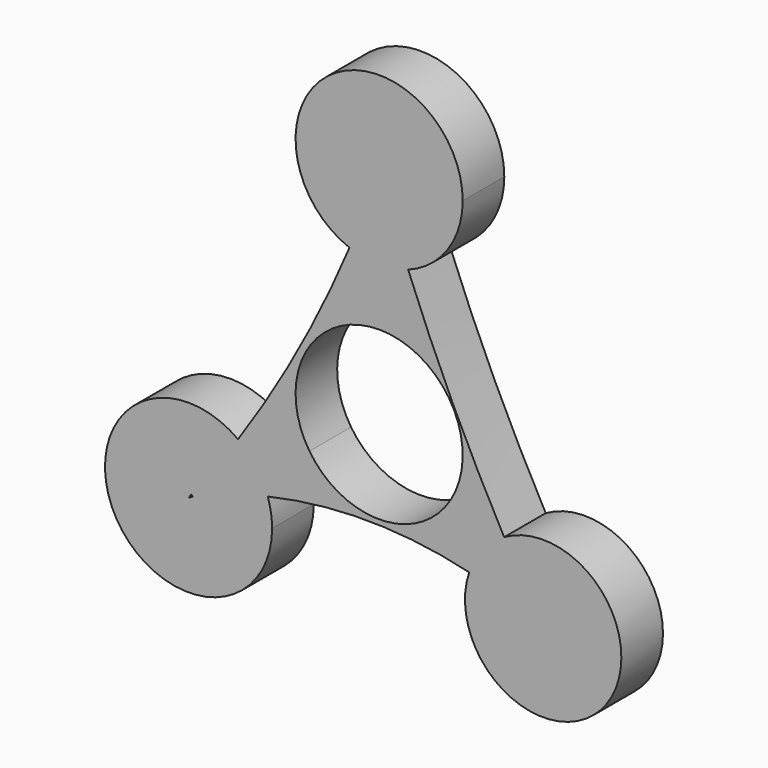
from build123d import *

# Parameters (mm, degrees)
F1_DEPTH = 7


with BuildPart() as f1:
    # F0 (on Front) → F1 (new body)
    with BuildSketch(Plane.XZ):
        with BuildLine():
            ThreePointArc((0, 11.25), (7.9549512883, 7.9549512883), (11.25, 0))
            ThreePointArc((11.25, 0), (10.6496799821, -3.625853869), (8.912788217, -6.8647437096))
            Line((8.912788217, -6.8647437096), (13.7440443636, -10.5858391104))
            ThreePointArc((13.7440443636, -10.5858391104), (15.1532765292, -9.0858880946), (16.8274285565, -7.8888069213))
            ThreePointArc((16.8274285565, -7.8888069213), (9.9384051979, 5.6621865141), (3.902940072, 19.6142912527))
            ThreePointArc((3.902940072, 19.6142912527), (1.9824951191, 19.091630603), (0, 18.9155735821))
            Line((0, 18.9155735821), (0, 11.25))
        make_face()
        with BuildLine():
            ThreePointArc((-9.3763874584, -6.216579303), (-9.9120890119, 5.3209953412), (0, 11.25))
            Line((0, 11.25), (0, 18.9155735821))
            ThreePointArc((0, 18.9155735821), (-2.0297975666, 19.1002031934), (-3.9929710023, 19.6480319218))
            ThreePointArc((-3.9929710023, 19.6480319218), (-10.8071521762, 5.4794924629), (-18.9966353601, -7.9411237916))
            ThreePointArc((-18.9966353601, -7.9411237916), (-17.5117499257, -9.2469886158), (-16.2784463054, -10.7926696541))
            Line((-16.2784463054, -10.7926696541), (-9.3763874584, -6.216579303))
        make_face()
        with BuildLine():
            Line((13.7440443636, -10.5858391104), (8.912788217, -6.8647437096))
            ThreePointArc((8.912788217, -6.8647437096), (-0.3984474102, -11.2429417708), (-9.3763874584, -6.216579303))
            Line((-9.3763874584, -6.216579303), (-16.2784463054, -10.7926696541))
            ThreePointArc((-16.2784463054, -10.7926696541), (-15.5501585, -12.0637421264), (-14.9932083314, -13.4186719648))
            ThreePointArc((-14.9932083314, -13.4186719648), (-1.4222887066, -11.9055225601), (12.1287440927, -13.58748292))
            ThreePointArc((12.1287440927, -13.58748292), (12.8140917314, -12.020845326), (13.7440443636, -10.5858391104))
        make_face()
        with BuildLine():
            Line((0, 30.1655735821), (0, 18.9155735821))
            ThreePointArc((0, 18.9155735821), (1.9824951191, 19.091630603), (3.902940072, 19.6142912527))
            ThreePointArc((3.902940072, 19.6142912527), (1.8909068472, 24.8675299748), (0, 30.1655735821))
        make_face()
        with BuildLine():
            ThreePointArc((-3.9929710023, 19.6480319218), (-2.0297975666, 19.1002031934), (0, 18.9155735821))
            Line((0, 18.9155735821), (0, 30.1655735821))
            ThreePointArc((0, 30.1655735821), (-1.902781485, 24.8712281442), (-3.9929710023, 19.6480319218))
        make_face()
        with BuildLine():
            Line((22.0838300884, -17.009248957), (13.7440443636, -10.5858391104))
            ThreePointArc((13.7440443636, -10.5858391104), (12.8140917314, -12.020845326), (12.1287440927, -13.58748292))
            ThreePointArc((12.1287440927, -13.58748292), (17.1835996068, -15.0734374251), (22.0838300884, -17.009248957))
        make_face()
        with BuildLine():
            ThreePointArc((16.8274285565, -7.8888069213), (15.1532765292, -9.0858880946), (13.7440443636, -10.5858391104))
            Line((13.7440443636, -10.5858391104), (22.0838300884, -17.009248957))
            ThreePointArc((22.0838300884, -17.009248957), (19.4066454, -12.4772589354), (16.8274285565, -7.8888069213))
        make_face()
        with BuildLine():
            Line((-25.1416982942, -16.6690382571), (-16.2784463054, -10.7926696541))
            ThreePointArc((-16.2784463054, -10.7926696541), (-17.5117499257, -9.2469886158), (-18.9966353601, -7.9411237916))
            ThreePointArc((-18.9966353601, -7.9411237916), (-22.0531670318, -12.2727527283), (-25.2533971823, -16.4993260556))
            ThreePointArc((-25.2533971823, -16.4993260556), (-25.19769062, -16.5842761963), (-25.1416982942, -16.6690382571))
        make_face()
        with BuildLine():
            ThreePointArc((-14.9932083314, -13.4186719648), (-15.5501585, -12.0637421264), (-16.2784463054, -10.7926696541))
            Line((-16.2784463054, -10.7926696541), (-25.1416982942, -16.6690382571))
            ThreePointArc((-25.1416982942, -16.6690382571), (-25.1125512398, -16.7129171531), (-25.0833276051, -16.7567450833))
            ThreePointArc((-25.0833276051, -16.7567450833), (-20.114417639, -14.8575280476), (-14.9932083314, -13.4186719648))
        make_face()
        with BuildLine():
            ThreePointArc((11.25, 30.1655735821), (-6.3891148144, 39.425255644), (-3.9929710023, 19.6480319218))
            ThreePointArc((-3.9929710023, 19.6480319218), (-1.902781485, 24.8712281442), (0, 30.1655735821))
            ThreePointArc((0, 30.1655735821), (1.8909068472, 24.8675299748), (3.902940072, 19.6142912527))
            ThreePointArc((3.902940072, 19.6142912527), (9.2322959173, 23.7369491495), (11.25, 30.1655735821))
        make_face()
        with BuildLine():
            ThreePointArc((32.6105684243, -17.009248957), (27.3506819222, -7.8948377444), (16.8274285565, -7.8888069213))
            ThreePointArc((16.8274285565, -7.8888069213), (19.4066454, -12.4772589354), (22.0838300884, -17.009248957))
            ThreePointArc((22.0838300884, -17.009248957), (17.1835996068, -15.0734374251), (12.1287440927, -13.58748292))
            ThreePointArc((12.1287440927, -13.58748292), (20.3492358123, -27.3920907015), (32.6105684243, -17.009248957))
        make_face()
        with BuildLine():
            ThreePointArc((-14.4048337638, -17.009248957), (-14.5529018122, -15.1900164424), (-14.9932083314, -13.4186719648))
            ThreePointArc((-14.9932083314, -13.4186719648), (-20.114417639, -14.8575280476), (-25.0833276051, -16.7567450833))
            ThreePointArc((-25.0833276051, -16.7567450833), (-25.3694186196, -16.8822321528), (-25.6548337638, -17.009248957))
            ThreePointArc((-25.6548337638, -17.009248957), (-25.4538534807, -16.7544937597), (-25.2533971823, -16.4993260556))
            ThreePointArc((-25.2533971823, -16.4993260556), (-22.0531670318, -12.2727527283), (-18.9966353601, -7.9411237916))
            ThreePointArc((-18.9966353601, -7.9411237916), (-35.6914475365, -22.0914614653), (-14.4048337638, -17.009248957))
        make_face()
    extrude(amount=F1_DEPTH)


solid = f1.part
